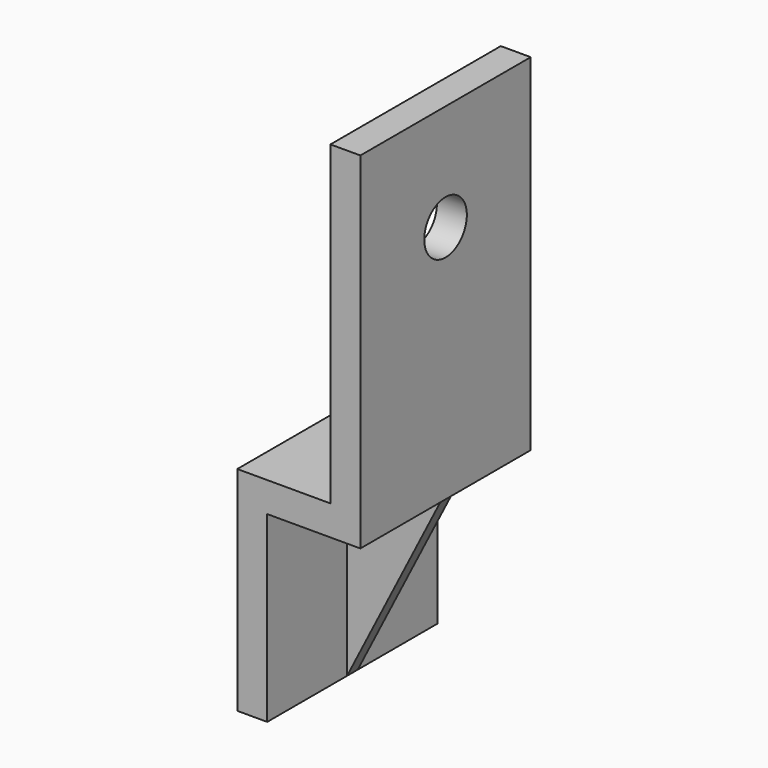
from build123d import *

# Parameters (mm, degrees)
F1_DEPTH  = 101.6
F3_D      = 25.4
F4_W      = 101.6
F4_H      = 87.3125
F5_DEPTH  = 44.45
F7_DEPTH  = 101.601
F8_W      = 47.625
F8_H      = 97.9758906887
F9_DEPTH  = 127.2487635172
F10_DEPTH = 127.2487635172


with BuildPart() as f1:
    # F0 (on Front) → F1 (new body)
    with BuildSketch(Plane.XZ):
        Polygon((-37.8673051461, 7.5604184782), (-37.8673051461, -94.0395815218), (-23.5798051461, -94.0395815218), (-23.5798051461, -6.7270815218), (20.8701948539, -6.7270815218), (20.8701948539, 158.3729184782), (6.5826948539, 158.3729184782), (6.5826948539, 7.5604184782), align=None)
    extrude(amount=F1_DEPTH)

    # F3 (through all)
    with Locations(Plane.YZ.offset(20.8701948539)):
        with Locations((-50.8, 107.5729184782)):
            Hole(F3_D / 2)


with BuildPart() as f5:
    # F4 (on face) → F5 (new body, through all)
    with BuildSketch(Plane.YZ.offset(-23.5798051461)):
        with Locations((-50.8, -50.3833315218)):
            Rectangle(F4_W, F4_H)
    extrude(amount=F5_DEPTH)

    # F6 (on face) → F7 (cut, through all)
    with BuildSketch(Plane.XZ.offset(101.6)):
        Polygon((20.8701948539, -6.7270815218), (-23.5798051461, -94.0395815218), (20.8701948539, -94.0395815218), align=None)
    extrude(amount=-F7_DEPTH, mode=Mode.SUBTRACT)

    # F8 (on face) → F9 (cut, through all)
    with BuildSketch(Plane(origin=(19.2943147747, 0, -9.8225602489), x_dir=(0, 1, 0), z_dir=(0.8911631156, 0, -0.4536830407))):
        with Locations((-23.8125, -45.5144188116)):
            Rectangle(F8_W, F8_H)
    extrude(amount=-F9_DEPTH, mode=Mode.SUBTRACT)

    # F8 (on face) → F10 (cut, through all)
    with BuildSketch(Plane(origin=(19.2943147747, 0, -9.8225602489), x_dir=(0, 1, 0), z_dir=(0.8911631156, 0, -0.4536830407))):
        with Locations((-77.7875, -45.5144188116)):
            Rectangle(F8_W, F8_H)
    extrude(amount=-F10_DEPTH, mode=Mode.SUBTRACT)


solid = Compound([f1.part, f5.part])
